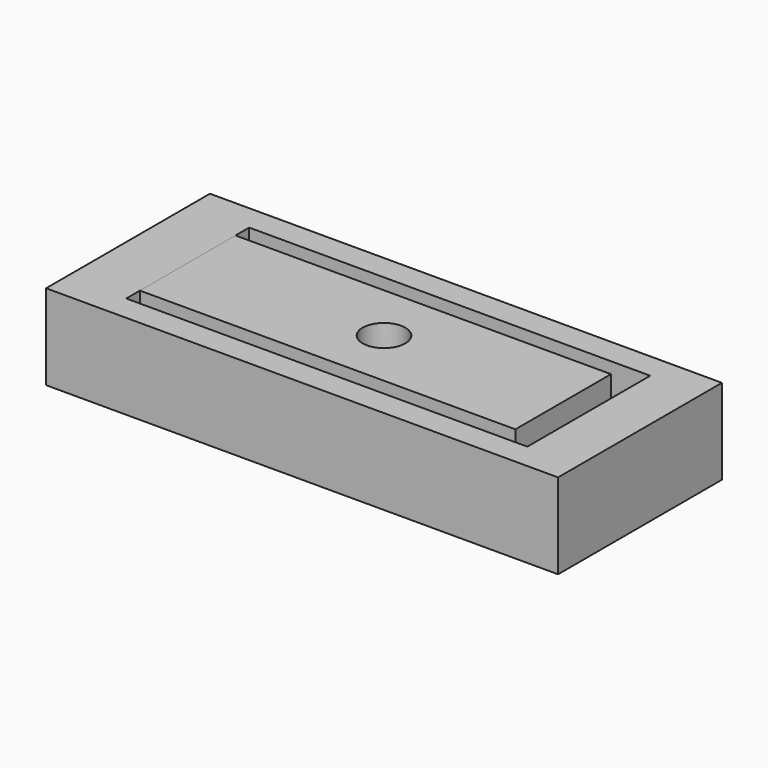
from build123d import *

# Parameters (mm, degrees)
F0_W      = 30
F0_H      = 12
F1_DEPTH  = 5
F2_T      = -1.5
F3_W      = 2
F3_H      = 9
F4_DEPTH  = 1.4
F5_W      = 1
F5_H      = 9
F6_DEPTH  = 3.5
F8_DEPTH  = 1.501
F9_W      = 1.5
F9_H      = 9
F10_DEPTH = 1.4
F11_SIZE2 = 1.39999
F11_SIZE  = 0.99999
F12_W     = 22
F12_H     = 7
F12_R     = 1.25
F13_DEPTH = 1.5
F15_DEPTH = 7
F17_DEPTH = 7


# Not quite as in the source:
# - a fillet or chamfer is up to 0.001 mm smaller than in the source, because OpenCascade refuses the exact size


with BuildPart() as f1:
    # F0 (on Top) → F1 (new body)
    with BuildSketch(Plane.XY):
        Rectangle(F0_W, F0_H)
    extrude(amount=F1_DEPTH)

    # F2
    f2_openings = [f1.faces().sort_by_distance(p)[0] for p in [
        (0, 0, 5),
    ]]
    offset(amount=F2_T, openings=f2_openings)

    # F3 (on face) → F4 (join)
    with BuildSketch(Plane.XY.offset(5)):
        with Locations((-12.5, 0)):
            Rectangle(F3_W, F3_H)
    extrude(amount=-F4_DEPTH)

    # F5 (on face) → F6 (join, through all)
    with BuildSketch(Plane.XY.offset(5)):
        with Locations((13, 0)):
            Rectangle(F5_W, F5_H)
    extrude(amount=-F6_DEPTH)

    # F7 (on face) → F8 (cut, through all)
    with BuildSketch(Plane.XY.offset(1.5)):
        with BuildLine():
            Line((5, 1.5), (-5, 1.5))
            ThreePointArc((-5, 1.5), (-5.7071067812, 1.2071067812), (-6, 0.5))
            Line((-6, 0.5), (-6, -0.5))
            ThreePointArc((-6, -0.5), (-5.7071067812, -1.2071067812), (-5, -1.5))
            Line((-5, -1.5), (5, -1.5))
            ThreePointArc((5, -1.5), (5.7071067812, -1.2071067812), (6, -0.5))
            Line((6, -0.5), (6, 0.5))
            ThreePointArc((6, 0.5), (5.7071067812, 1.2071067812), (5, 1.5))
        make_face()
    extrude(amount=-F8_DEPTH, mode=Mode.SUBTRACT)

    # F9 (on face) → F10 (join)
    with BuildSketch(Plane.XY.offset(5)):
        with Locations((11.75, 0)):
            Rectangle(F9_W, F9_H)
    extrude(amount=-F10_DEPTH)

    # F11 (size 1 and 1.4 in the source; OpenCascade refuses exactly that, so slightly less here)
    f11_edges = [f1.edges().sort_by_distance(p)[0] for p in [
        (11, 0, 5),
    ]]
    f11_side = f1.faces().sort_by_distance((0, 5.67689, 5))[0]
    chamfer(f11_edges, length=F11_SIZE, length2=F11_SIZE2, reference=f11_side)


with BuildPart() as f13:
    # F12 (on face) → F13 (new body)
    with BuildSketch(Plane.XY.offset(5)):
        with Locations((-0.5, 0)):
            Rectangle(F12_W, F12_H)
        Circle(F12_R, mode=Mode.SUBTRACT)
    extrude(amount=-F13_DEPTH)

    # F14 (on face) → F15 (join, through all)
    with BuildSketch(Plane.XZ.offset(3.5)):
        Polygon((-8.5, 3.5), (-11.5, 3.5), (-11.5, 3.1), (-12.5, 3.1), (-12.5, 2), (-8.5, 2), align=None)
    extrude(amount=-F15_DEPTH)

    # F16 (on face) → F17 (join, through all)
    with BuildSketch(Plane.XZ.offset(3.5)):
        Polygon((10.5, 3.1), (10.5, 3.5), (8, 3.5), (8, 2), (11.5, 2), (11.5, 3.1), align=None)
    extrude(amount=-F17_DEPTH)


solid = Compound([f1.part, f13.part])
